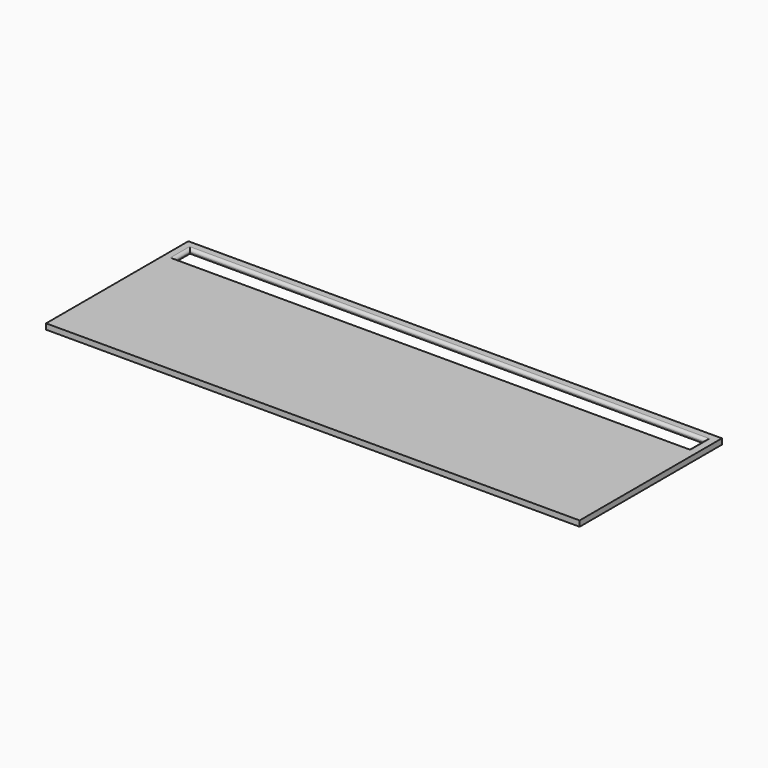
from build123d import *

# Parameters (mm, degrees)
F0_W     = 190.5
F0_H     = 63.5
F1_DEPTH = 2
F2_W     = 183.896
F2_H     = 7.62
F3_DEPTH = 25.4
F4_R     = 0.99999
F5_R     = 0.99999


# Not quite as in the source:
# - a fillet or chamfer is up to 0.001 mm smaller than in the source, because OpenCascade refuses the exact size


with BuildPart() as f1:
    # F0 (on Top) → F1 (new body)
    with BuildSketch(Plane.XY):
        with Locations((1.791532172, 31.75)):
            Rectangle(F0_W, F0_H)
    extrude(amount=F1_DEPTH)

    # F2 (on face) → F3 (cut)
    with BuildSketch(Plane.XY.offset(2)):
        with Locations((1.791532172, 56.388)):
            Rectangle(F2_W, F2_H)
    extrude(amount=-F3_DEPTH, mode=Mode.SUBTRACT)

    # F4 (radius 1 in the source; OpenCascade refuses exactly that, so slightly less here)
    f4_edges = [f1.edges().sort_by_distance(p)[0] for p in [
        (1.791532, 60.198, 2),
        (1.791532, 60.198, 0),
    ]]
    fillet(f4_edges, radius=F4_R)

    # F5 (radius 1 in the source; OpenCascade refuses exactly that, so slightly less here)
    f5_edges = [f1.edges().sort_by_distance(p)[0] for p in [
        (93.739532, 56.388, 0),
        (93.739532, 56.388, 2),
        (-90.156468, 56.388, 2),
        (-90.156468, 56.388, 0),
    ]]
    fillet(f5_edges, radius=F5_R)


solid = f1.part
